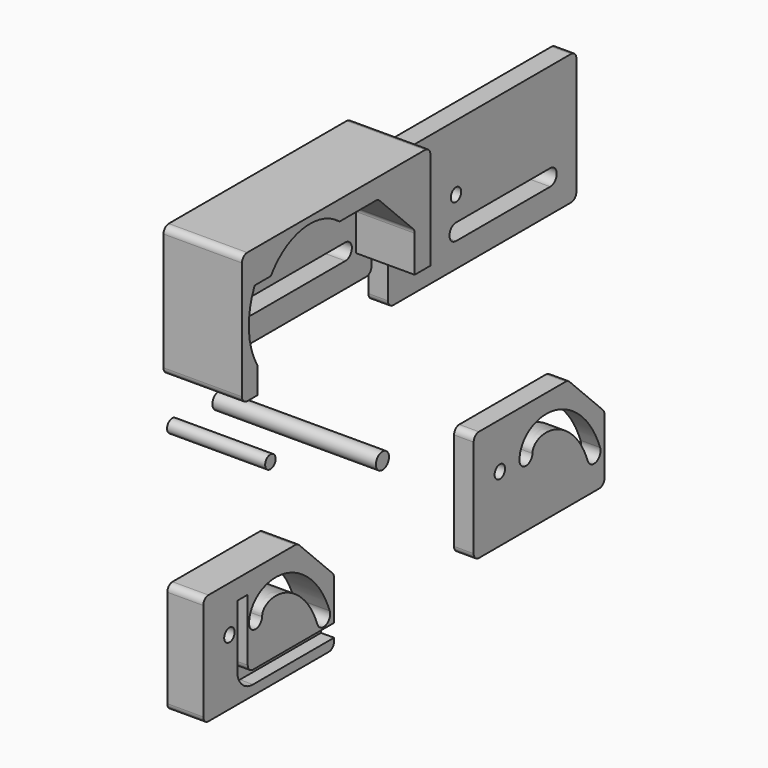
from build123d import *

# Parameters (mm, degrees)
F0_R      = 1
F1_DEPTH  = 3
F2_DEPTH  = 5.5
F3_DEPTH  = 15
F0_R_2    = 1.25
F4_DEPTH  = 25
F5_DEPTH  = 3
F7_DEPTH  = 2
F8_DEPTH  = 12
F9_R      = 1
F10_DEPTH = 9


# Not quite as in the source:
# - the dataset's text gives a spline's control points without its knots; the knots are read off the source's solid


with BuildPart() as f1:
    # F0 (on Right) → F1 (new body)
    with BuildSketch(Plane.YZ):
        with BuildLine():
            Line((-108.3511220217, 68.5771017373), (-142.3511220217, 68.5771017373))
            ThreePointArc((-142.3511220217, 68.5771017373), (-143.0582288029, 68.2842085184), (-143.3511220217, 67.5771017373))
            Line((-143.3511220217, 67.5771017373), (-143.3511220217, 49.5771017373))
            ThreePointArc((-143.3511220217, 49.5771017373), (-143.0582288029, 48.8699949561), (-142.3511220217, 48.5771017373))
            Line((-142.3511220217, 48.5771017373), (-108.3511220217, 48.5771017373))
            ThreePointArc((-108.3511220217, 48.5771017373), (-107.6440152405, 48.8699949561), (-107.3511220217, 49.5771017373))
            Line((-107.3511220217, 49.5771017373), (-107.3511220217, 67.5771017373))
            ThreePointArc((-107.3511220217, 67.5771017373), (-107.6440152405, 68.2842085184), (-108.3511220217, 68.5771017373))
        make_face()
        with BuildLine():
            Line((-112.3511220217, 52.3271017373), (-130.3511220217, 52.3271017373))
            ThreePointArc((-130.3511220217, 52.3271017373), (-131.6011220217, 53.5771017373), (-130.3511220217, 54.8271017373))
            Line((-130.3511220217, 54.8271017373), (-112.3511220217, 54.8271017373))
            ThreePointArc((-112.3511220217, 54.8271017373), (-111.1011220217, 53.5771017373), (-112.3511220217, 52.3271017373))
        make_face(mode=Mode.SUBTRACT)
        with Locations((-130.3511220217, 58.5771017373)):
            Circle(F0_R, mode=Mode.SUBTRACT)
    extrude(amount=F1_DEPTH)


with BuildPart() as f2:
    # F0 (on Right) → F2 (new body)
    with BuildSketch(Plane.YZ):
        with BuildLine():
            ThreePointArc((-181.7793399096, 9.9999977499), (-181.4864466907, 9.2928909687), (-180.7793399096, 8.9999977499))
            Line((-180.7793399096, 8.9999977499), (-157.7793399096, 8.9999977499))
            ThreePointArc((-157.7793399096, 8.9999977499), (-157.0722331284, 9.2928909687), (-156.7793399096, 9.9999977499))
            Line((-156.7793399096, 9.9999977499), (-156.7793399096, 18.5857841876))
            ThreePointArc((-156.7793399096, 18.5857841876), (-156.855460377, 18.9684676199), (-157.0722331284, 19.2928909687))
            Line((-157.0722331284, 19.2928909687), (-163.4864466907, 25.7071045311))
            ThreePointArc((-163.4864466907, 25.7071045311), (-163.8108700396, 25.9238772824), (-164.1935534719, 25.9999977499))
            Line((-164.1935534719, 25.9999977499), (-180.7793399096, 25.9999977499))
            ThreePointArc((-180.7793399096, 25.9999977499), (-181.4864466907, 25.7071045311), (-181.7793399096, 24.9999977499))
            Line((-181.7793399096, 24.9999977499), (-181.7793399096, 9.9999977499))
        make_face()
        with Locations((-176.7793399096, 18.9999977499)):
            Circle(F0_R, mode=Mode.SUBTRACT)
        with BuildLine():
            add(Edge.make_bspline(
                [(-170.5324331908, 18.9121134937), (-170.5299731128, 18.9470172177), (-170.5253464114, 19.0125013809), (-170.518407998, 19.0975741515), (-170.5110063987, 19.1692953385), (-170.5030826553, 19.2275845694), (-170.497013985, 19.2612777736), (-170.4930944874, 19.2798514111), (-170.490576774, 19.2910355206), (-170.4869459981, 19.3057574492), (-170.4817927424, 19.3244518788), (-170.4737972413, 19.3507509342), (-170.456747093, 19.4001960165), (-170.4331774108, 19.4558522137), (-170.4082803674, 19.5066912539), (-170.3903568801, 19.5415181497), (-170.3665546726, 19.5846362487), (-170.3358518354, 19.6354873808), (-170.2920123222, 19.7021144151), (-170.2437901293, 19.7668943278), (-170.1911418923, 19.8296253122), (-170.1343828975, 19.8922416502), (-170.0560855495, 19.9695671495), (-169.95078166, 20.0596879291), (-169.796124043, 20.1747033707), (-169.576951309, 20.3069263955), (-169.2755151857, 20.4416779233), (-168.9393394251, 20.5483637985), (-168.4507157584, 20.6484723801), (-167.7762478252, 20.6877849718), (-166.8997564401, 20.5860049652), (-165.9877306, 20.3323809753), (-165.067236682, 19.9292591852), (-164.3122217509, 19.4734520149), (-163.7252733414, 19.0408607651), (-163.295815632, 18.6835858054), (-162.8786109354, 18.2943501137), (-162.475848935, 17.8748271472), (-162.1541155047, 17.5012895905), (-161.9061600842, 17.1888821575), (-161.6638588696, 16.8665637722), (-161.4302822088, 16.5301110832), (-161.2052773552, 16.1799016004), (-161.0419217248, 15.9122905268), (-160.8853667211, 15.6409782094), (-160.7359309099, 15.3655692545), (-160.6176402341, 15.1322932677), (-160.5273365943, 14.9440423922), (-160.438680545, 14.7519842747), (-160.3296928871, 14.5033601032), (-160.1579415144, 14.0900025819), (-160.0298951998, 13.764498324), (-159.942650452, 13.5426045035)],
                knots=[0, 0, 0, 0, 0.0078125, 0.015625, 0.0234375, 0.03125, 0.0390625, 0.041015625, 0.04296875, 0.046875, 0.05078125, 0.0546875, 0.0625, 0.078125, 0.08203125, 0.0859375, 0.09375, 0.1015625, 0.109375, 0.125, 0.1328125, 0.140625, 0.15625, 0.171875, 0.1875, 0.21875, 0.25, 0.28125, 0.3125, 0.375, 0.4375, 0.5, 0.5625, 0.625, 0.65625, 0.6875, 0.71875, 0.75, 0.78125, 0.796875, 0.8125, 0.84375, 0.859375, 0.875, 0.890625, 0.90625, 0.921875, 0.9296875, 0.9375, 0.953125, 0.96875, 1, 1, 1, 1], degree=3))
            ThreePointArc((-170.5324331908, 18.9121134937), (-171.8672241628, 17.7530910344), (-173.0262466221, 19.0878820064))
            add(Edge.make_bspline(
                [(-173.0262466221, 19.0878820064), (-173.0237865443, 19.1227857268), (-173.0185729288, 19.1969164522), (-173.0085847676, 19.3209329621), (-172.9947274076, 19.4576349477), (-172.9748942298, 19.6067697381), (-172.9536455814, 19.7276453702), (-172.9359708577, 19.8115972604), (-172.9231401971, 19.8686177156), (-172.9057658486, 19.9388659803), (-172.8829069338, 20.0216436673), (-172.8499300972, 20.1299371755), (-172.7860948858, 20.3140579451), (-172.71170594, 20.4875277806), (-172.6422873637, 20.6292014873), (-172.5947039028, 20.7216329598), (-172.5067185881, 20.8810157466), (-172.3674221571, 21.1019361348), (-172.2105786444, 21.3125626376), (-172.0748158928, 21.4742634431), (-171.9335878251, 21.6299516304), (-171.7471570969, 21.8137014526), (-171.5093002986, 22.0169129272), (-171.1752949835, 22.2649398536), (-170.7294944073, 22.5323608494), (-170.1594647606, 22.7858648418), (-169.5633896116, 22.9739575334), (-168.7435138184, 23.1407903096), (-167.6862347706, 23.1985248174), (-166.404057416, 23.0465240906), (-165.13659606, 22.6918232344), (-163.9065880986, 22.151432604), (-162.9283781698, 21.5597453329), (-162.1815025929, 21.0091007337), (-161.6409219491, 20.559232332), (-161.1217240919, 20.0747013388), (-160.6248279102, 19.5570161693), (-160.2303130841, 19.09893209), (-159.9271483078, 18.7169362254), (-159.6332905637, 18.3259984261), (-159.3530332625, 17.9221196169), (-159.0864805344, 17.507230754), (-158.8923231766, 17.1891910726), (-158.7038761801, 16.8626789103), (-158.5221390102, 16.5277684575), (-158.3770688009, 16.2417683212), (-158.2649422833, 16.0080126766), (-158.1567981924, 15.7736812612), (-158.0290687829, 15.4820776156), (-157.8369627635, 15.01946156), (-157.7032741149, 14.6792848168), (-157.6160293671, 14.4573909963)],
                knots=[0, 0, 0, 0, 0.0078125, 0.015625, 0.0234375, 0.03125, 0.0390625, 0.041015625, 0.04296875, 0.046875, 0.05078125, 0.0546875, 0.0625, 0.078125, 0.08203125, 0.0859375, 0.09375, 0.109375, 0.125, 0.1328125, 0.140625, 0.15625, 0.171875, 0.1875, 0.21875, 0.25, 0.28125, 0.3125, 0.375, 0.4375, 0.5, 0.5625, 0.625, 0.65625, 0.6875, 0.71875, 0.75, 0.78125, 0.796875, 0.8125, 0.84375, 0.859375, 0.875, 0.890625, 0.90625, 0.921875, 0.9296875, 0.9375, 0.953125, 0.96875, 1, 1, 1, 1], degree=3))
            ThreePointArc((-157.6160293671, 14.4573909963), (-158.3219466631, 12.8366872075), (-159.942650452, 13.5426045035))
        make_face(mode=Mode.SUBTRACT)
    extrude(amount=F2_DEPTH)

    # F6 (on face) → F7 (cut)
    with BuildSketch(Plane.YZ.offset(5.5)):
        with BuildLine():
            Line((-172.2793399096, 10.4999977499), (-156.7793399096, 10.4999977499))
            Line((-156.7793399096, 10.4999977499), (-156.7793399096, 12.4999977499))
            Line((-156.7793399096, 12.4999977499), (-172.2793399096, 12.4999977499))
            ThreePointArc((-172.2793399096, 12.4999977499), (-172.9864466907, 12.7928909687), (-173.2793399096, 13.4999977499))
            Line((-173.2793399096, 13.4999977499), (-173.2793399096, 22.9999977499))
            Line((-173.2793399096, 22.9999977499), (-175.2793399096, 22.9999977499))
            Line((-175.2793399096, 22.9999977499), (-175.2793399096, 13.4999977499))
            ThreePointArc((-175.2793399096, 13.4999977499), (-174.4006602531, 11.3786774064), (-172.2793399096, 10.4999977499))
        make_face()
    extrude(amount=-F7_DEPTH, mode=Mode.SUBTRACT)


with BuildPart() as f3:
    # F0 (on Right) → F3 (new body)
    with BuildSketch(Plane.YZ):
        with Locations((-180.8265447617, 47.0357015729)):
            Circle(F0_R)
    extrude(amount=F3_DEPTH)


with BuildPart() as f4:
    # F0 (on Right) → F4 (new body)
    with BuildSketch(Plane.YZ):
        with Locations((-171.9105690718, 46.8103773892)):
            Circle(F0_R_2)
    extrude(amount=F4_DEPTH)


with BuildPart() as f5:
    # F0 (on Right) → F5 (new body)
    with BuildSketch(Plane.YZ):
        with BuildLine():
            ThreePointArc((-126.975330159, 8.888440731), (-126.6824369402, 8.1813339498), (-125.975330159, 7.888440731))
            Line((-125.975330159, 7.888440731), (-102.975330159, 7.888440731))
            ThreePointArc((-102.975330159, 7.888440731), (-102.2682233778, 8.1813339498), (-101.975330159, 8.888440731))
            Line((-101.975330159, 8.888440731), (-101.975330159, 17.4742271686))
            ThreePointArc((-101.975330159, 17.4742271686), (-102.0514506265, 17.856910601), (-102.2682233778, 18.1813339498))
            Line((-102.2682233778, 18.1813339498), (-108.6824369402, 24.5955475122))
            ThreePointArc((-108.6824369402, 24.5955475122), (-109.006860289, 24.8123202635), (-109.3895437214, 24.888440731))
            Line((-109.3895437214, 24.888440731), (-125.975330159, 24.888440731))
            ThreePointArc((-125.975330159, 24.888440731), (-126.6824369402, 24.5955475122), (-126.975330159, 23.888440731))
            Line((-126.975330159, 23.888440731), (-126.975330159, 8.888440731))
        make_face()
        with BuildLine():
            add(Edge.make_bspline(
                [(-115.7284234578, 17.8005564787), (-115.7259633805, 17.835460192), (-115.7213366795, 17.9009443369), (-115.714398265, 17.9860170894), (-115.7069966636, 18.0577382678), (-115.6990729175, 18.1160274997), (-115.6930042446, 18.1497207123), (-115.6890847446, 18.1682943584), (-115.6865670294, 18.1794784746), (-115.6829362513, 18.1942004108), (-115.6777829931, 18.2128948482), (-115.6697874891, 18.2391939124), (-115.6527373369, 18.288639006), (-115.6291676537, 18.3442952061), (-115.604270612, 18.3951342441), (-115.5863471265, 18.4299611369), (-115.562544921, 18.4730792327), (-115.5318420854, 18.5239303622), (-115.4880025735, 18.5905573943), (-115.4397803805, 18.655337307), (-115.3871321422, 18.7180682927), (-115.3303731465, 18.7806846316), (-115.2520757979, 18.8580101313), (-115.1467719086, 18.9481309108), (-114.9921142922, 19.0631463519), (-114.772941558, 19.1953693768), (-114.4715054346, 19.3301209046), (-114.135329674, 19.4368067798), (-113.6467060073, 19.5369153613), (-112.972238074, 19.5762279529), (-112.095746689, 19.4744479462), (-111.183720849, 19.2208239562), (-110.263226931, 18.8177021661), (-109.508212, 18.3618949957), (-108.9212635905, 17.9293037459), (-108.4918058811, 17.5720287862), (-108.0746011846, 17.1827930945), (-107.6718391843, 16.7632701281), (-107.350105754, 16.3897325714), (-107.1021503335, 16.0773251384), (-106.8598491189, 15.7550067531), (-106.6262724581, 15.4185540642), (-106.4012676046, 15.0683445814), (-106.2379119741, 14.8007335077), (-106.0813569705, 14.5294211904), (-105.9319211593, 14.2540122355), (-105.8136304835, 14.0207362487), (-105.7233268437, 13.8324853732), (-105.6346707944, 13.6404272557), (-105.5256831366, 13.3918030842), (-105.3539317638, 12.978445563), (-105.2258854492, 12.6529413051), (-105.1386407014, 12.4310474846)],
                knots=[0, 0, 0, 0, 0.0078125, 0.015625, 0.0234375, 0.03125, 0.0390625, 0.041015625, 0.04296875, 0.046875, 0.05078125, 0.0546875, 0.0625, 0.078125, 0.08203125, 0.0859375, 0.09375, 0.1015625, 0.109375, 0.125, 0.1328125, 0.140625, 0.15625, 0.171875, 0.1875, 0.21875, 0.25, 0.28125, 0.3125, 0.375, 0.4375, 0.5, 0.5625, 0.625, 0.65625, 0.6875, 0.71875, 0.75, 0.78125, 0.796875, 0.8125, 0.84375, 0.859375, 0.875, 0.890625, 0.90625, 0.921875, 0.9296875, 0.9375, 0.953125, 0.96875, 1, 1, 1, 1], degree=3))
            ThreePointArc((-115.7284234578, 17.8005564787), (-117.0632144298, 16.6415340194), (-118.2222368891, 17.9763249914))
            add(Edge.make_bspline(
                [(-118.2222368891, 17.9763249914), (-118.2197768106, 18.0112287224), (-118.2145631928, 18.0853594658), (-118.2045750265, 18.2093759927), (-118.19071766, 18.3460779856), (-118.1708844759, 18.4952127732), (-118.1496358242, 18.6160883959), (-118.1319610997, 18.700040277), (-118.1191304392, 18.7570607253), (-118.1017560911, 18.8273089821), (-118.0788971774, 18.9100866609), (-118.0459203427, 19.0183801601), (-117.9820851353, 19.2025009185), (-117.9076961928, 19.3759707515), (-117.8382776168, 19.5176444606), (-117.790694155, 19.6100759364), (-117.7027088385, 19.7694587277), (-117.5634124051, 19.9903791192), (-117.4065688914, 20.201005622), (-117.2708061405, 20.362706426), (-117.1295780735, 20.5183946123), (-116.9431473459, 20.7021444339), (-116.7052905476, 20.9053559086), (-116.371285232, 21.1533828354), (-115.9254846557, 21.420803831), (-115.3554550092, 21.6743078232), (-114.7593798601, 21.8624005147), (-113.9395040669, 22.0292332908), (-112.8822250192, 22.0869677984), (-111.6000476647, 21.9349670715), (-110.3325863088, 21.5802662152), (-109.1025783474, 21.0398755848), (-108.1243684187, 20.4481883136), (-107.3774928419, 19.8975437145), (-106.8369121981, 19.4476753128), (-106.317714341, 18.9631443196), (-105.8208181594, 18.4454591501), (-105.4263033333, 17.9873750708), (-105.1231385571, 17.6053792063), (-104.829280813, 17.214441407), (-104.5490235118, 16.8105625978), (-104.2824707837, 16.3956737349), (-104.088313426, 16.0776340535), (-103.8998664295, 15.7511218912), (-103.7181292595, 15.4162114384), (-103.5730590503, 15.1302113021), (-103.4609325327, 14.8964556576), (-103.3527884418, 14.6621242422), (-103.2250590323, 14.3705205966), (-103.0329530129, 13.9079045411), (-102.8992643644, 13.5677277979), (-102.8120196165, 13.3458339774)],
                knots=[0, 0, 0, 0, 0.0078125, 0.015625, 0.0234375, 0.03125, 0.0390625, 0.041015625, 0.04296875, 0.046875, 0.05078125, 0.0546875, 0.0625, 0.078125, 0.08203125, 0.0859375, 0.09375, 0.109375, 0.125, 0.1328125, 0.140625, 0.15625, 0.171875, 0.1875, 0.21875, 0.25, 0.28125, 0.3125, 0.375, 0.4375, 0.5, 0.5625, 0.625, 0.65625, 0.6875, 0.71875, 0.75, 0.78125, 0.796875, 0.8125, 0.84375, 0.859375, 0.875, 0.890625, 0.90625, 0.921875, 0.9296875, 0.9375, 0.953125, 0.96875, 1, 1, 1, 1], degree=3))
            ThreePointArc((-102.8120196165, 13.3458339774), (-103.5179369126, 11.7251301886), (-105.1386407014, 12.4310474846))
        make_face(mode=Mode.SUBTRACT)
        with Locations((-121.975330159, 17.888440731)):
            Circle(F0_R, mode=Mode.SUBTRACT)
    extrude(amount=F5_DEPTH)


with BuildPart() as f8:
    # F0 (on Right) → F8 (new body)
    with BuildSketch(Plane.YZ):
        with BuildLine():
            Line((-147.5008541346, 74.5035414398), (-181.5008541346, 74.5035414398))
            ThreePointArc((-181.5008541346, 74.5035414398), (-182.2079609157, 74.210648221), (-182.5008541346, 73.5035414398))
            Line((-182.5008541346, 73.5035414398), (-182.5008541346, 55.5035414398))
            ThreePointArc((-182.5008541346, 55.5035414398), (-182.2079609157, 54.7964346586), (-181.5008541346, 54.5035414398))
            Line((-181.5008541346, 54.5035414398), (-147.5008541346, 54.5035414398))
            ThreePointArc((-147.5008541346, 54.5035414398), (-146.7937473534, 54.7964346586), (-146.5008541346, 55.5035414398))
            Line((-146.5008541346, 55.5035414398), (-146.5008541346, 73.5035414398))
            ThreePointArc((-146.5008541346, 73.5035414398), (-146.7937473534, 74.210648221), (-147.5008541346, 74.5035414398))
        make_face()
        with BuildLine():
            Line((-151.5008541346, 58.2535414398), (-169.5008541346, 58.2535414398))
            ThreePointArc((-169.5008541346, 58.2535414398), (-170.7508541346, 59.5035414398), (-169.5008541346, 60.7535414398))
            Line((-169.5008541346, 60.7535414398), (-151.5008541346, 60.7535414398))
            ThreePointArc((-151.5008541346, 60.7535414398), (-150.2508541346, 59.5035414398), (-151.5008541346, 58.2535414398))
        make_face(mode=Mode.SUBTRACT)
        with Locations((-169.5008541346, 64.5035414398)):
            Circle(F0_R, mode=Mode.SUBTRACT)
    extrude(amount=F8_DEPTH)

    # F9 (on face) → F10 (cut)
    with BuildSketch(Plane.YZ.offset(12)):
        with BuildLine():
            Line((-146.5008541346, 55.5035414398), (-146.5008541346, 58.5035414398))
            Line((-146.5008541346, 58.5035414398), (-149.5008541346, 58.5035414398))
            Line((-149.5008541346, 58.5035414398), (-149.5008541346, 64.0893278774))
            ThreePointArc((-149.5008541346, 64.0893278774), (-149.576974602, 64.4720113098), (-149.7937473534, 64.7964346586))
            Line((-149.7937473534, 64.7964346586), (-156.2079609157, 71.210648221))
            ThreePointArc((-156.2079609157, 71.210648221), (-156.5323842646, 71.4274209723), (-156.9150676969, 71.5035414398))
            Line((-156.9150676969, 71.5035414398), (-163.8439998851, 71.5035414398))
            ThreePointArc((-163.8439998851, 71.5035414398), (-170.8551028235, 73.4010697757), (-176.9841689081, 69.5035414398))
            Line((-176.9841689081, 69.5035414398), (-180.0786610906, 69.5035414398))
            ThreePointArc((-180.0786610906, 69.5035414398), (-181.1849595526, 63.8938853231), (-179.5008541346, 58.4298275841))
            Line((-179.5008541346, 58.4298275841), (-179.5008541346, 54.5035414398))
            Line((-179.5008541346, 54.5035414398), (-147.5008541346, 54.5035414398))
            ThreePointArc((-147.5008541346, 54.5035414398), (-146.7937473534, 54.7964346586), (-146.5008541346, 55.5035414398))
        make_face()
        with BuildLine():
            Line((-169.5008541346, 60.7535414398), (-151.5008541346, 60.7535414398))
            ThreePointArc((-151.5008541346, 60.7535414398), (-150.2508541346, 59.5035414398), (-151.5008541346, 58.2535414398))
            Line((-151.5008541346, 58.2535414398), (-169.5008541346, 58.2535414398))
            ThreePointArc((-169.5008541346, 58.2535414398), (-170.7508541346, 59.5035414398), (-169.5008541346, 60.7535414398))
        make_face(mode=Mode.SUBTRACT)
        with Locations((-169.5008541346, 64.5035414398)):
            Circle(F9_R, mode=Mode.SUBTRACT)
    extrude(amount=-F10_DEPTH, mode=Mode.SUBTRACT)


solid = Compound([f1.part, f2.part, f3.part, f4.part, f5.part, f8.part])
